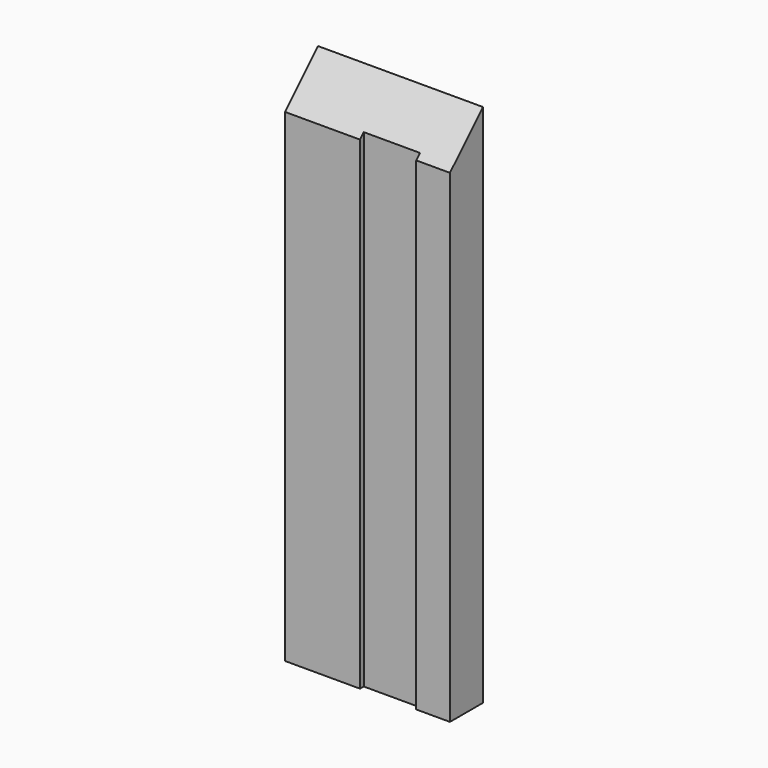
from build123d import *

# Parameters (mm, degrees)
F0_W     = 111.76
F0_H     = 27.94
F1_DEPTH = 355.6
F2_SIZE  = 27.93999
F3_W     = 38.1
F3_H     = 27.93999
F3_H_2   = 327.66001
F4_DEPTH = 3.175


# Not quite as in the source:
# - a fillet or chamfer is up to 0.001 mm smaller than in the source, because OpenCascade refuses the exact size


with BuildPart() as f1:
    # F0 (on Top) → F1 (new body)
    with BuildSketch(Plane.XY):
        with Locations((55.88, -13.97)):
            Rectangle(F0_W, F0_H)
    extrude(amount=F1_DEPTH)

    # F2 (size 27.94 in the source; OpenCascade refuses exactly that, so slightly less here)
    f2_edges = [f1.edges().sort_by_distance(p)[0] for p in [
        (55.88, -27.94, 355.6),
    ]]
    chamfer(f2_edges, length=F2_SIZE)

    # F3 (on face) → F4 (cut)
    with BuildSketch(Plane.XZ.offset(27.94)):
        with Locations((69.85, 341.630005)):
            Rectangle(F3_W, F3_H)
        with Locations((69.85, 163.830005)):
            Rectangle(F3_W, F3_H_2)
    extrude(amount=-F4_DEPTH, mode=Mode.SUBTRACT)


solid = f1.part
